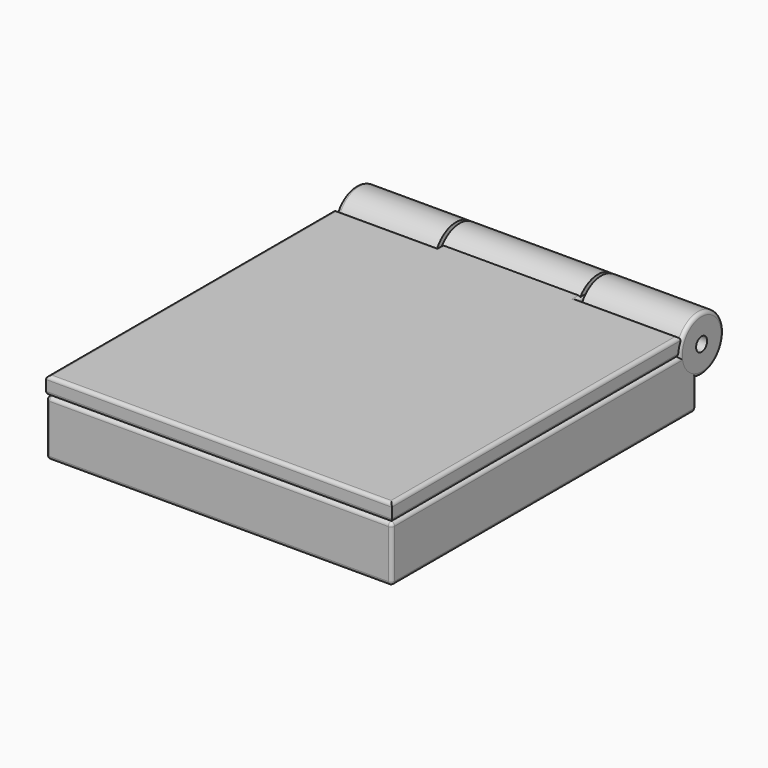
from build123d import *

# Parameters (mm, degrees)
F0_R          = 4
F0_R_2        = 1
F3_DEPTH      = 10
F3_DEPTH_BACK = 10
F2_W          = 55
F2_H          = 2.5
F4_DEPTH      = 25
F4_DEPTH_BACK = 25
F1_W          = 55
F1_H          = 8
F5_W          = 20.5
F5_H          = 4.125
F6_DEPTH      = 5
F8_R          = 4
F8_R_2        = 1
F9_DEPTH      = 14.5
F11_R         = 4.25
F12_DEPTH     = 14.8
F13_R         = 4.25
F14_DEPTH     = 14.8
F15_T         = 2.5
F15_T3_DEPTH  = 10
F15_T5_DEPTH  = 9.125
F15_T7_DEPTH  = 25.5
F18_R         = 3
F19_DEPTH     = 5.5
F20_R         = 1.9
F21_DEPTH     = 2
F22_R         = 0.5
F22_2_R       = 0.5
F22_3_R       = 0.5
F23_R         = 0.5
F24_R         = 1.9
F25_DEPTH     = 1.8


# Not quite as in the source:
# - a shell that OpenCascade refuses in one call is made with other operations: the cavity is built on its own and cut out


with BuildPart() as f3:
    # F0 (on Right) → F3 (new body, two sides)
    with BuildSketch(Plane.YZ) as f3_sk:
        Circle(F0_R)
        Circle(F0_R_2, mode=Mode.SUBTRACT)
    extrude(amount=F3_DEPTH)
    extrude(f3_sk.sketch, amount=-F3_DEPTH_BACK)


with BuildPart() as f4:
    # F2 (on Right) → F4 (new body, two sides)
    with BuildSketch(Plane.YZ) as f4_sk:
        with Locations((-28.5, 1.25)):
            Rectangle(F2_W, F2_H)
    extrude(amount=F4_DEPTH)
    extrude(f4_sk.sketch, amount=-F4_DEPTH_BACK)

    # F11 (on face) → F12 (cut)
    with BuildSketch(Plane.YZ.offset(25)):
        Circle(F11_R)
    extrude(amount=-F12_DEPTH, mode=Mode.SUBTRACT)

    # F13 (on face) → F14 (cut)
    with BuildSketch(Plane(origin=(-25, 0, 0), x_dir=(0, -1, 0), z_dir=(-1, 0, 0))):
        Circle(F13_R)
    extrude(amount=-F14_DEPTH, mode=Mode.SUBTRACT)

    # F23
    f23_edges = [f4.edges().sort_by_distance(p)[0] for p in [
        (10.2, -2.218466, 2.5),
        (0, -1, 2.5),
        (-10.2, -2.218466, 2.5),
        (-17.6, -3.436932, 2.5),
        (-25, -29.718466, 2.5),
        (0, -56, 2.5),
        (25, -29.718466, 2.5),
        (17.6, -3.436932, 2.5),
        (0, -56, 0),
        (-25, -30.125, 0),
        (-17.6, -4.25, 0),
        (-10.2, -2.625, 0),
        (0, -1, 0),
        (10.2, -2.625, 0),
        (17.6, -4.25, 0),
        (25, -30.125, 0),
    ]]
    fillet(f23_edges, radius=F23_R)

    # F24 (on face) → F25 (cut)
    with BuildSketch(Plane(origin=(0, 0, 0), x_dir=(1, 0, 0), z_dir=(0, 0, -1))):
        with Locations((21.5, 52.4921567416)):
            Circle(F24_R)
        with Locations((-21.5, 52.4921567416)):
            Circle(F24_R)
    extrude(amount=-F25_DEPTH, mode=Mode.SUBTRACT)


with BuildPart() as f4b:
    # F1 (on Right) → F4, piece 2 (new body, two sides)
    with BuildSketch(Plane.YZ) as f4_2_sk:
        with Locations((-28.4921567416, -4.125)):
            Rectangle(F1_W, F1_H)
    extrude(amount=F4_DEPTH)
    extrude(f4_2_sk.sketch, amount=-F4_DEPTH_BACK)

    # F5 (on face) → F6 (cut)
    with BuildSketch(Plane(origin=(0, -0.9921567416, 0), x_dir=(-1, 0, 0), z_dir=(0, 1, 0))):
        with Locations((0, -2.1875)):
            Rectangle(F5_W, F5_H)
    extrude(amount=-F6_DEPTH, mode=Mode.SUBTRACT)

    # F15: shell of thickness 2.5, made by hand


with BuildPart() as f9:
    # F8 (on offset) → F9 (new body, through all)
    with BuildSketch(Plane.YZ.offset(10.5)):
        Circle(F8_R)
        Circle(F8_R_2, mode=Mode.SUBTRACT)
    extrude(amount=F9_DEPTH)


with BuildPart() as f10_1:
    # F10: instance of F9
    add(f9.part.mirror(Plane.YZ))

    # F22#3
    f22_3_edges = [f10_1.edges().sort_by_distance(p)[0] for p in [
        (-25, -4, 0),
    ]]
    fillet(f22_3_edges, radius=F22_3_R)


with BuildPart() as f15_core1:
    # F15_t2: copy of F4b
    add(f4b.part)

    # the walls: a layer under each face that stays
    f15_faces = [f15_core1.faces().sort_by_distance(p)[0] for p in [
        (16.6666666667, -0.9921567416, -6.7916666667),
        (0, -28.4921567416, -8.125),
        (-25, -28.4921567416, -4.125),
        (-10.25, -3.4921567416, -2.1875),
        (0, -3.4921567416, -4.25),
        (10.25, -3.4921567416, -2.1875),
        (25, -28.4921567416, -4.125),
        (0, -55.9921567416, -4.125),
        (0, -5.9921567416, -2.1875),
    ]]
    thicken(f15_faces, amount=-F15_T, mode=Mode.SUBTRACT)

    # F15_s4 → F15_t3 (cut)
    with BuildSketch(Plane.XZ.offset(-1.5078432584)):
        Polygon((-10.225, -4.225), (-12.75, -4.25), (-12.75, -6.75), (-10.25, -6.75), align=None)
        Polygon((10.225, -4.225), (10.25, -6.75), (12.75, -6.75), (12.75, -4.25), align=None)
    extrude(amount=F15_T3_DEPTH, mode=Mode.SUBTRACT)

    # F15_s6 → F15_t5 (cut)
    with BuildSketch(Plane.XY.offset(-6.75)):
        Polygon((-10.225, -5.9671567416), (-12.75, -5.9921567416), (-12.75, -8.4921567416), (-10.25, -8.4921567416), align=None)
        Polygon((10.225, -5.9671567416), (12.75, -5.9921567416), (12.75, -8.4921567416), (10.25, -8.4921567416), align=None)
    extrude(amount=F15_T5_DEPTH, mode=Mode.SUBTRACT)

    # F15_s8 → F15_t7 (cut)
    with BuildSketch(Plane.YZ.offset(-12.75)):
        Polygon((-5.9671567416, -4.225), (-5.9921567416, -6.75), (-8.4921567416, -6.75), (-8.4921567416, -4.25), align=None)
    extrude(amount=F15_T7_DEPTH, mode=Mode.SUBTRACT)


with BuildPart() as f4b_1:
    add(f4b.part)

    # what is left inside the walls is the cavity
    f15_cavity = [f15_core1.part.solids().sort_by_distance(p)[0] for p in [
        (7.5, -28.492157, -5.6),
    ]]
    add(f15_cavity, mode=Mode.SUBTRACT)

    # F18 (on offset) → F19 (join, through all)
    with BuildSketch(Plane.XY.offset(-0.125)):
        with Locations((-21.5, -52.4921567416)):
            Circle(F18_R)
        with Locations((21.5, -52.4921567416)):
            Circle(F18_R)
    extrude(amount=-F19_DEPTH)

    # F20 (on offset) → F21 (cut)
    with BuildSketch(Plane.XY.offset(-0.125)):
        with Locations((-21.5, -52.4921567416)):
            Circle(F20_R)
        with Locations((21.5, -52.4921567416)):
            Circle(F20_R)
    extrude(amount=-F21_DEPTH, mode=Mode.SUBTRACT)

    # F22
    f22_edges = [f4b_1.edges().sort_by_distance(p)[0] for p in [
        (0, -53.492157, -5.625),
        (19.37868, -50.370836, -5.625),
        (22.5, -26.577943, -5.625),
        (17.625, -3.492157, -5.625),
        (12.75, -5.992157, -5.625),
        (11.494431, -8.492157, -5.625),
        (0, -8.492157, -5.625),
        (-11.494431, -8.492157, -5.625),
        (-12.75, -5.992157, -5.625),
        (-17.625, -3.492157, -5.625),
        (-22.5, -26.577943, -5.625),
        (-19.37868, -50.370836, -5.625),
        (25, -55.992157, -4.125),
        (0, -55.992157, -8.125),
        (-25, -55.992157, -4.125),
        (0, -55.992157, -0.125),
        (25, -0.992157, -4.125),
        (25, -28.492157, -0.125),
        (25, -28.492157, -8.125),
        (-25, -0.992157, -4.125),
        (-25, -28.492157, -0.125),
        (-25, -28.492157, -8.125),
        (0, -0.992157, -8.125),
        (-22.5, -26.577943, -0.125),
        (-19.37868, -50.370836, -0.125),
        (0, -53.492157, -0.125),
        (19.37868, -50.370836, -0.125),
        (22.5, -26.577943, -0.125),
        (0, -8.492157, -0.125),
        (0, -5.992157, -0.125),
        (10.25, -3.492157, -0.125),
        (-10.25, -3.492157, -0.125),
        (-12.75, -5.992157, -0.125),
        (-11.5, -8.492157, -0.125),
        (11.5, -8.492157, -0.125),
        (12.75, -5.992157, -0.125),
    ]]
    fillet(f22_edges, radius=F22_R)


with BuildPart() as f9_1:
    add(f9.part)

    # F22#2
    f22_2_edges = [f9_1.edges().sort_by_distance(p)[0] for p in [
        (25, -4, 0),
    ]]
    fillet(f22_2_edges, radius=F22_2_R)


solid = Compound([f3.part, f4.part, f10_1.part, f4b_1.part, f9_1.part])
